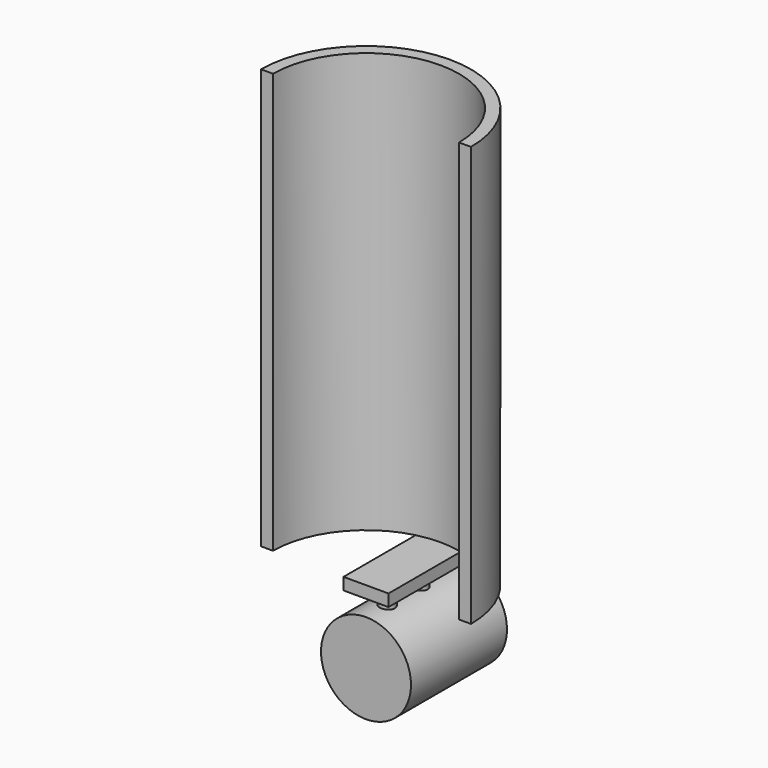
from build123d import *

# Parameters (mm, degrees)
F1_DEPTH = 88.9
F3_DEPTH = 2.54
F4_DEPTH = 25.4
F5_R     = 9.525
F6_DEPTH = 25.4
F7_R     = 1.5875
F8_DEPTH = 19.05


with BuildPart() as f1:
    # F0 (on Top) → F1 (new body)
    with BuildSketch(Plane.XY):
        with BuildLine():
            ThreePointArc((-19.685, 0), (0, 19.685), (19.685, 0))
            Line((19.685, 0), (22.225, 0))
            ThreePointArc((22.225, 0), (0, 22.225), (-22.225, 0))
            Line((-22.225, 0), (-19.685, 0))
        make_face()
    extrude(amount=F1_DEPTH)

    # F2 (on Top) → F3 (join)
    with BuildSketch(Plane.XY):
        Polygon((-4.7625, 22.2813114524), (-4.7625, 0), (4.7625, 0), (4.7625, 22.2813114524), (0, 22.2813114524), align=None)
        Polygon((-4.7625, 24.765), (-4.7625, 22.2813114524), (0, 22.2813114524), (4.7625, 22.2813114524), (4.7625, 24.765), align=None)
    extrude(amount=-F3_DEPTH)

    # F4 (add): a face of the model
    f4_faces = [f1.faces().sort_by_distance(p)[0] for p in [
        (0, 23.4050055059, 0),
    ]]
    extrude(f4_faces, amount=F4_DEPTH)

    # F7 (on Top) → F8 (join)
    with BuildSketch(Plane.XY):
        with Locations((0, 5.6055821072)):
            Circle(F7_R)
        with Locations((0, 14.2991673201)):
            Circle(F7_R)
    extrude(amount=-F8_DEPTH)


with BuildPart() as f6:
    # F5 (on Front) → F6 (new body)
    with BuildSketch(Plane.XZ):
        with Locations((0, -15.4736751718)):
            Circle(F5_R)
    extrude(amount=-F6_DEPTH)


solid = Compound([f1.part, f6.part])
